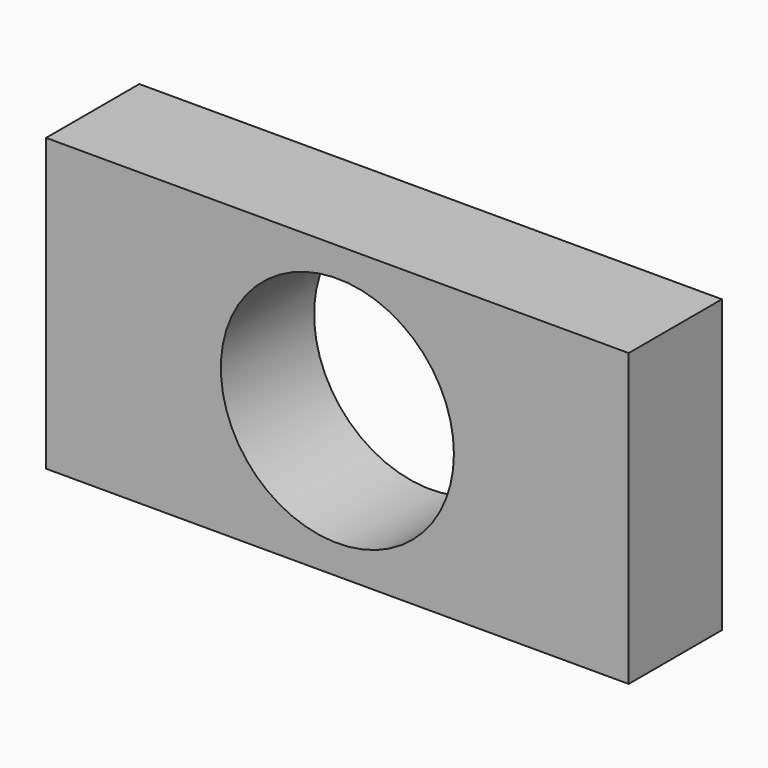
from build123d import *

# Parameters (mm, degrees)
F0_W     = 254
F0_H     = 127
F0_R     = 50.8
F1_DEPTH = 50.8


# Not quite as in the source:
# - a feature names something its author has since deleted; it is built from what else it names


with BuildPart() as f1:
    # F0 (on Front) → F1 (new body)
    with BuildSketch(Plane.XZ):
        Rectangle(F0_W, F0_H)
        Circle(F0_R, mode=Mode.SUBTRACT)
    extrude(amount=F1_DEPTH)


solid = f1.part
